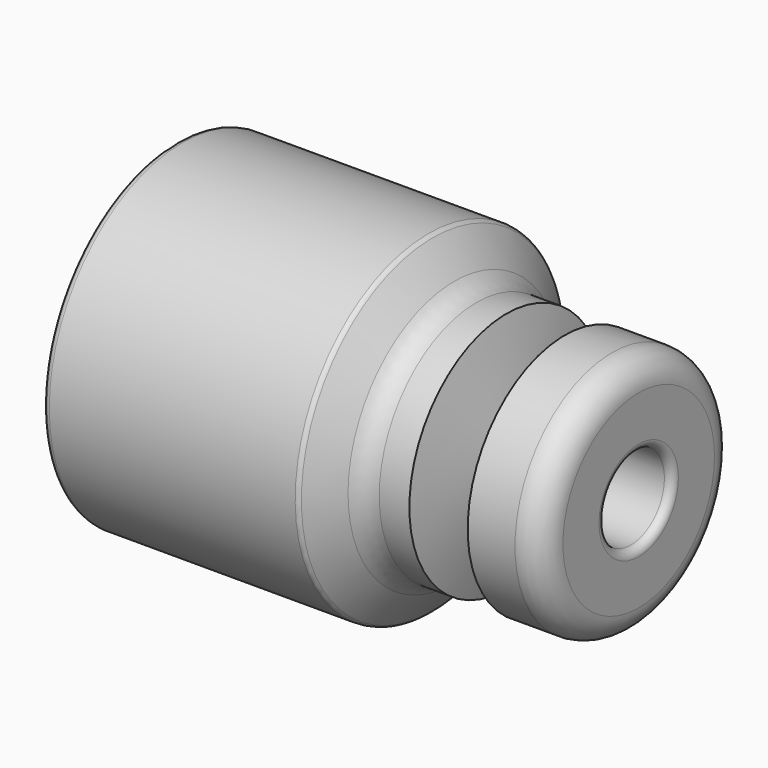
from build123d import *

# Parameters (mm, degrees)
F2_R     = 2.5527
F3_DEPTH = 25.4
F4_R     = 0.508
F5_R     = 2.54


# Not quite as in the source:
# - a feature names something its author has since deleted; it is built from what else it names


with BuildPart() as f1:
    # F0 (on Top) → F1 (revolve)
    with BuildSketch(Plane.XY):
        with BuildLine():
            ThreePointArc((-12.7, 5.2578), (-12.3280256121, 4.3597743879), (-11.43, 3.9878))
            Line((-11.43, 3.9878), (21.59, 3.9878))
            Line((21.59, 3.9878), (30.6736943138, 3.9878))
            ThreePointArc((30.6736943138, 3.9878), (31.1964370123, 4.2043271153), (31.4129641276, 4.7270698138))
            Line((31.4129641276, 4.7270698138), (31.4129641276, 11.2707641276))
            Line((31.4129641276, 11.2707641276), (31.4129641276, 11.5681612351))
            Line((31.4129641276, 11.5681612351), (24.3683144, 11.5681612351))
            Line((24.3683144, 11.5681612351), (22.86, 5.2578))
            Line((22.86, 5.2578), (21.59, 5.2578))
            Line((21.59, 5.2578), (20.32, 5.2578))
            Line((20.32, 5.2578), (18.8103442021, 11.5681612351))
            Line((18.8103442021, 11.5681612351), (14.6019718679, 11.5681612351))
            Line((14.6019718679, 11.5681612351), (11.638822034, 15.875))
            Line((11.638822034, 15.875), (-12.065, 15.875))
            ThreePointArc((-12.065, 15.875), (-12.5140128061, 15.6890128061), (-12.7, 15.24))
            Line((-12.7, 15.24), (-12.7, 5.2578))
        make_face()
    revolve(axis=Axis((0.6358246983, 0, 0), (1, 0, 0)))

    # F2 (on Top) → F3 (cut)
    with BuildSketch(Plane.XY):
        Circle(F2_R)
    extrude(amount=-F3_DEPTH, mode=Mode.SUBTRACT)

    # F4
    f4_edges = [f1.edges().sort_by_distance(p)[0] for p in [
        (-0.213089, 15.875, 0),
        (-12.065, -15.875, 0),
        (11.638822, -15.875, 0),
        (-2.5527, 0, -15.875),
    ]]
    fillet(f4_edges, radius=F4_R)

    # F5
    f5_edges = [f1.edges().sort_by_distance(p)[0] for p in [
        (31.412964, -11.568161, 0),
        (14.601972, -11.568161, 0),
    ]]
    fillet(f5_edges, radius=F5_R)


solid = f1.part
